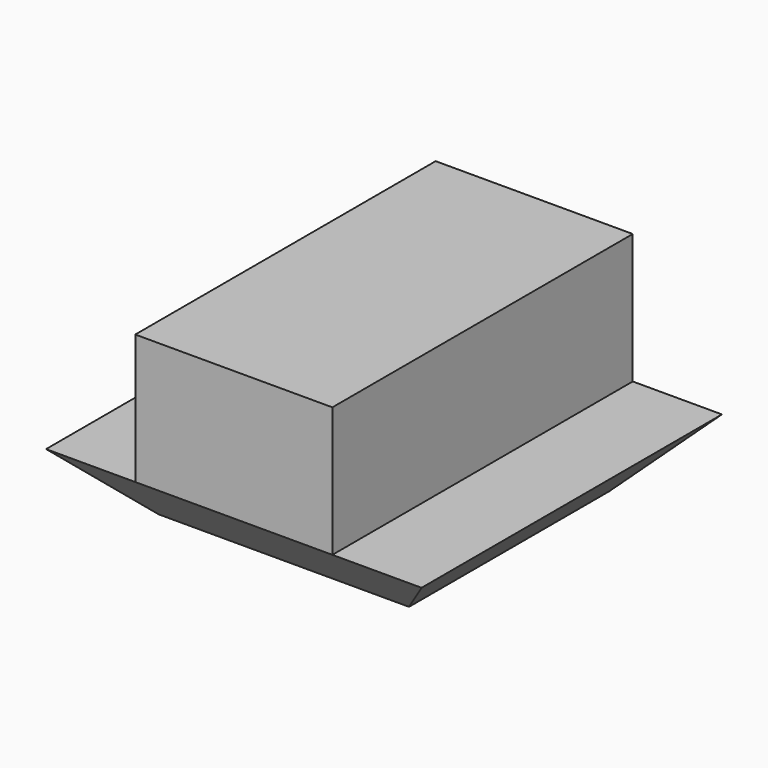
from build123d import *

# Parameters (mm, degrees)
F0_W     = 12
F0_H     = 12
F1_DEPTH = 2
F2_W     = 6.3
F2_H     = 12
F3_DEPTH = 4.15
F4_SIZE  = 1.99999


# Not quite as in the source:
# - a fillet or chamfer is up to 0.001 mm smaller than in the source, because OpenCascade refuses the exact size


with BuildPart() as f1:
    # F0 (on Top) → F1 (new body)
    with BuildSketch(Plane.XY):
        Rectangle(F0_W, F0_H)
    extrude(amount=F1_DEPTH)

    # F2 (on face) → F3 (join)
    with BuildSketch(Plane.XY.offset(2)):
        Rectangle(F2_W, F2_H)
    extrude(amount=F3_DEPTH)

    # F4 (size 2 in the source; OpenCascade refuses exactly that, so slightly less here)
    f4_edges = [f1.edges().sort_by_distance(p)[0] for p in [
        (6, 0, 0),
        (0, -6, 0),
        (-6, 0, 0),
        (0, 6, 0),
    ]]
    chamfer(f4_edges, length=F4_SIZE)


solid = f1.part
